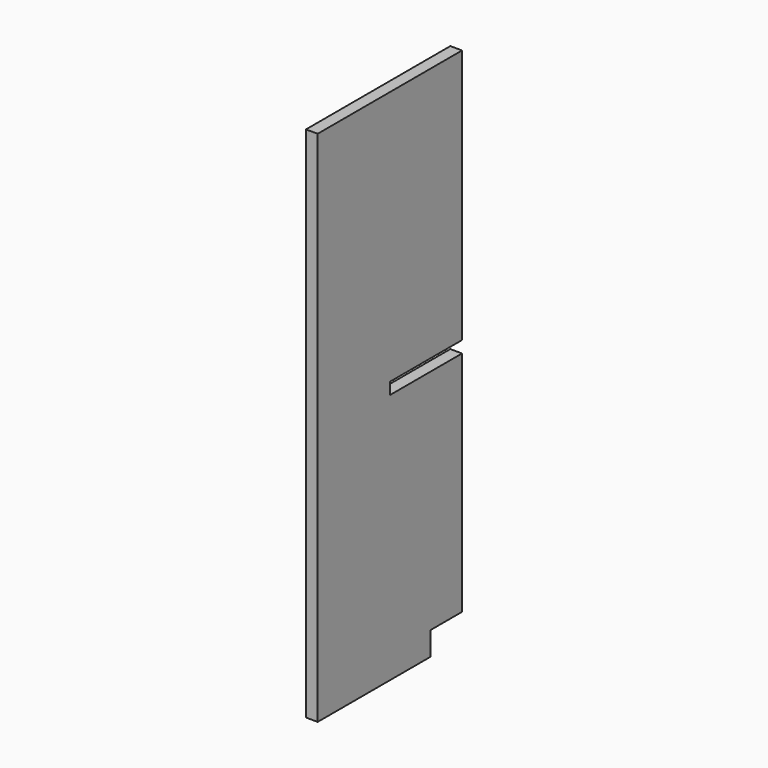
from build123d import *

# Parameters (mm, degrees)
F0_W     = 146.05
F0_H     = 412.75
F0_H_2   = 406.4
F0_H_3   = 19.05
F1_DEPTH = 19.05


with BuildPart() as f1:
    # F0 (on Right) → F1 (new body)
    with BuildSketch(Plane.YZ):
        with Locations((-73.025, 212.725)):
            Rectangle(F0_W, F0_H)
        with Locations((73.025, 212.725)):
            Rectangle(F0_W, F0_H)
        Polygon((146.05, -12.7), (0, -12.7), (0, -419.1), (82.55, -419.1), (82.55, -381), (146.05, -381), align=None)
        with Locations((-73.025, -215.9)):
            Rectangle(F0_W, F0_H_2)
        with Locations((-73.025, -3.175)):
            Rectangle(F0_W, F0_H_3)
    extrude(amount=F1_DEPTH)


solid = f1.part
